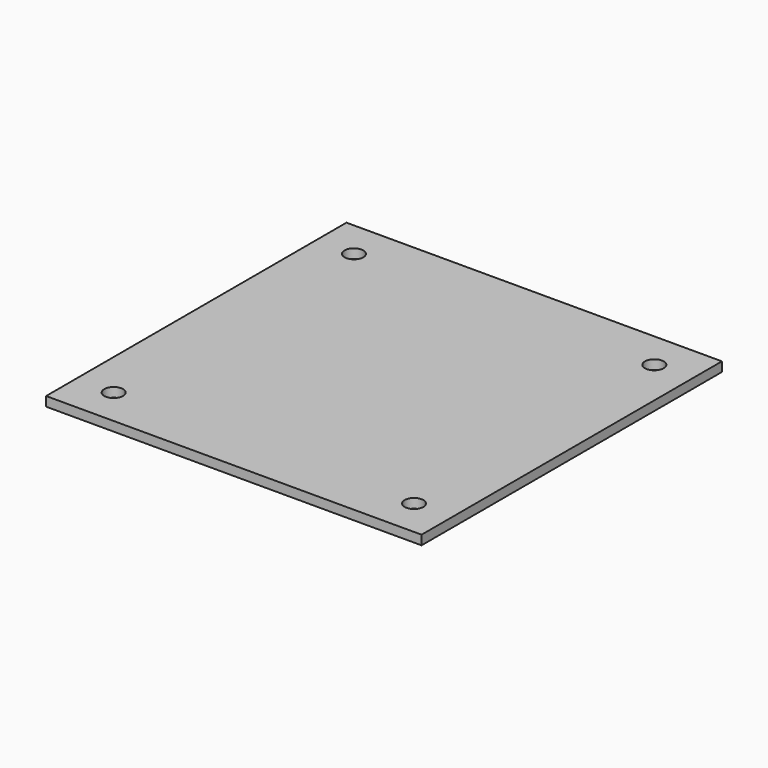
from build123d import *

# Parameters (mm, degrees)
F0_W     = 254
F0_H     = 254
F1_DEPTH = 6.35
F2_R     = 6.35
F3_DEPTH = 12.7
F4_DEPTH = 6.351


# Not quite as in the source:
# - a feature names something its author has since deleted; it is built from what else it names


with BuildPart() as f1:
    # F0 (on Top) → F1 (new body)
    with BuildSketch(Plane.XY):
        Rectangle(F0_W, F0_H)
    extrude(amount=F1_DEPTH)

    # F2 (on face) → F3 (cut)
    with BuildSketch(Plane.XY.offset(6.35)):
        with Locations((-101.6, 101.6)):
            Circle(F2_R)
        with Locations((-101.6, -101.6)):
            Circle(F2_R)
        with Locations((101.6, 101.6)):
            Circle(F2_R)
        with Locations((101.6, -101.6)):
            Circle(F2_R)
    extrude(amount=-F3_DEPTH, mode=Mode.SUBTRACT)

    # F2 (on face) → F4 (cut, through all)
    with BuildSketch(Plane.XY.offset(6.35)):
        with Locations((-101.6, 101.6)):
            Circle(F2_R)
        with Locations((-101.6, -101.6)):
            Circle(F2_R)
        with Locations((101.6, 101.6)):
            Circle(F2_R)
        with Locations((101.6, -101.6)):
            Circle(F2_R)
    extrude(amount=-F4_DEPTH, mode=Mode.SUBTRACT)


solid = f1.part
